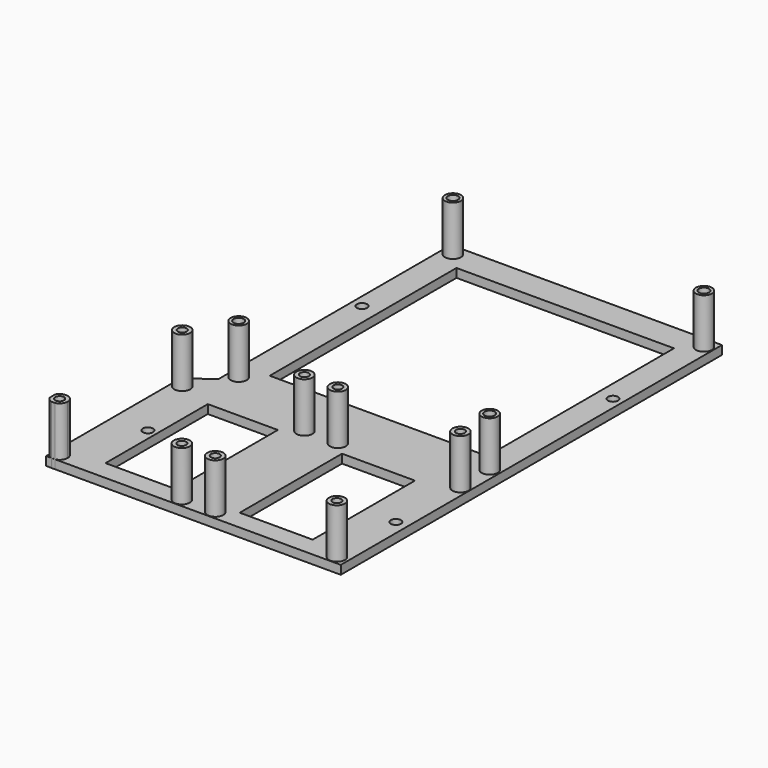
from build123d import *

# Parameters (mm, degrees)
F0_R     = 1.5
F0_R_2   = 1.75
F0_R_3   = 2.75
F0_W     = 24
F0_H     = 43.8174021336
F0_W_2   = 25
F0_W_3   = 74.5545638204
F0_H_2   = 80
F1_DEPTH = 3
F2_DEPTH = 20
F3_DEPTH = 20


# Not quite as in the source:
# - a feature names something its author has since deleted; it is built from what else it names


with BuildPart() as f1:
    # F0 (on Top) → F1 (new body)
    with BuildSketch(Plane.XY):
        with BuildLine():
            ThreePointArc((-47.6736667828, -81.2138915062), (-46.0983603754, -80.2573488478), (-45.4808032601, -78.5209193664))
            ThreePointArc((-45.4808032601, -78.5209193664), (-47.6409939689, -75.8349139681), (-50.7278032601, -77.3687514099))
            Line((-50.7278032601, -77.3687514099), (-50.7278032601, -79.6730873229))
            ThreePointArc((-50.7278032601, -79.6730873229), (-49.9411999358, -80.6742988526), (-48.7879397374, -81.2138915062))
            Line((-48.7879397374, -81.2138915062), (-47.6736667828, -81.2138915062))
        make_face()
        with Locations((-48.2308032601, -78.5209193664)):
            Circle(F0_R, mode=Mode.SUBTRACT)
        with BuildLine():
            ThreePointArc((-50.7278032601, -77.3687514099), (-47.6409939689, -75.8349139681), (-45.4808032601, -78.5209193664))
            ThreePointArc((-45.4808032601, -78.5209193664), (-46.0983603754, -80.2573488478), (-47.6736667828, -81.2138915062))
            Line((-47.6736667828, -81.2138915062), (50.2721967399, -81.2138915062))
            Line((50.2721967399, -81.2138915062), (50.3258705139, 82))
            Line((50.3258705139, 82), (-42.5516068935, 82))
            Line((-42.5516068935, 82), (-42.5516068935, -17.5))
            Line((-42.5516068935, -17.5), (-50.7278032601, -23.6660409719))
            Line((-50.7278032601, -23.6660409719), (-50.7278032601, -77.3687514099))
        make_face()
        with Locations((-38.7351833579, -52.5912989332)):
            Circle(F0_R_2, mode=Mode.SUBTRACT)
        with Locations((-6.5308032601, -78.3)):
            Circle(F0_R_3, mode=Mode.SUBTRACT)
        with Locations((-23.7278032601, -52.5912989332)):
            Rectangle(F0_W, F0_H, mode=Mode.SUBTRACT)
        with Locations((-47.5, -26.9212964922)):
            Circle(F0_R_3, mode=Mode.SUBTRACT)
        with Locations((-38.9970433209, -13.3562097783)):
            Circle(F0_R_3, mode=Mode.SUBTRACT)
        with Locations((-5.8, -26.7)):
            Circle(F0_R_3, mode=Mode.SUBTRACT)
        with Locations((4.9221967399, -78.3)):
            Circle(F0_R_3, mode=Mode.SUBTRACT)
        with Locations((22.7721967399, -52.5912989332)):
            Rectangle(F0_W_2, F0_H, mode=Mode.SUBTRACT)
        with Locations((46.6221967399, -78.3)):
            Circle(F0_R_3, mode=Mode.SUBTRACT)
        with Locations((46.2721967399, -52.5912989332)):
            Circle(F0_R_2, mode=Mode.SUBTRACT)
        with Locations((5.6529477609, -26.7)):
            Circle(F0_R_3, mode=Mode.SUBTRACT)
        with Locations((47.3529477609, -26.2951753209)):
            Circle(F0_R_3, mode=Mode.SUBTRACT)
        with Locations((47.0029571713, -13.3550426021)):
            Circle(F0_R_3, mode=Mode.SUBTRACT)
        with Locations((-38.9970430732, 39.4713241122)):
            Circle(F0_R_2, mode=Mode.SUBTRACT)
        with Locations((-38.7351833579, 78.1026230454)):
            Circle(F0_R_3, mode=Mode.SUBTRACT)
        with Locations((4.2256750166, 32.5)):
            Rectangle(F0_W_3, F0_H_2, mode=Mode.SUBTRACT)
        with Locations((47.0029569268, 39.4713241122)):
            Circle(F0_R_2, mode=Mode.SUBTRACT)
        with Locations((47.2648166418, 78.1026230454)):
            Circle(F0_R_3, mode=Mode.SUBTRACT)
        with BuildLine():
            Line((-50.7278032601, -79.6730873229), (-50.7278032601, -77.3687514099))
            ThreePointArc((-50.7278032601, -77.3687514099), (-50.9808032601, -78.5209193664), (-50.7278032601, -79.6730873229))
        make_face()
        with BuildLine():
            ThreePointArc((-48.7879397374, -81.2138915062), (-48.2308032601, -81.2709193664), (-47.6736667828, -81.2138915062))
            Line((-47.6736667828, -81.2138915062), (-48.7879397374, -81.2138915062))
        make_face()
        with BuildLine():
            ThreePointArc((-48.7879397374, -81.2138915062), (-49.9411999358, -80.6742988526), (-50.7278032601, -79.6730873229))
            Line((-50.7278032601, -79.6730873229), (-50.7278032601, -81.2138915062))
            Line((-50.7278032601, -81.2138915062), (-48.7879397374, -81.2138915062))
        make_face()
    extrude(amount=F1_DEPTH)

    # F0 (on Top) → F2 (join)
    with BuildSketch(Plane.XY):
        with Locations((-38.7351833579, 78.1026230454)):
            Circle(F0_R_3)
        with Locations((-38.7351833579, 78.1026230454)):
            Circle(F0_R_2, mode=Mode.SUBTRACT)
    extrude(amount=F2_DEPTH)

    # F0 (on Top) → F3 (join)
    with BuildSketch(Plane.XY):
        with Locations((47.2648166418, 78.1026230454)):
            Circle(F0_R_3)
        with Locations((47.2648166418, 78.1026230454)):
            Circle(F0_R_2, mode=Mode.SUBTRACT)
        with Locations((-38.9970433209, -13.3562097783)):
            Circle(F0_R_3)
        with Locations((-38.9970433209, -13.3562097783)):
            Circle(F0_R_2, mode=Mode.SUBTRACT)
        with Locations((47.3529477609, -26.2951753209)):
            Circle(F0_R_3)
        with Locations((47.3529477609, -26.2951753209)):
            Circle(F0_R, mode=Mode.SUBTRACT)
        with Locations((5.6529477609, -26.7)):
            Circle(F0_R_3)
        with Locations((5.6529477609, -26.7)):
            Circle(F0_R, mode=Mode.SUBTRACT)
        with Locations((-5.8, -26.7)):
            Circle(F0_R_3)
        with Locations((-5.8, -26.7)):
            Circle(F0_R, mode=Mode.SUBTRACT)
        with Locations((-47.5, -26.9212964922)):
            Circle(F0_R_3)
        with Locations((-47.5, -26.9212964922)):
            Circle(F0_R, mode=Mode.SUBTRACT)
        with BuildLine():
            ThreePointArc((-47.6736667828, -81.2138915062), (-46.0983603754, -80.2573488478), (-45.4808032601, -78.5209193664))
            ThreePointArc((-45.4808032601, -78.5209193664), (-47.6409939689, -75.8349139681), (-50.7278032601, -77.3687514099))
            Line((-50.7278032601, -77.3687514099), (-50.7278032601, -79.6730873229))
            ThreePointArc((-50.7278032601, -79.6730873229), (-49.9411999358, -80.6742988526), (-48.7879397374, -81.2138915062))
            Line((-48.7879397374, -81.2138915062), (-47.6736667828, -81.2138915062))
        make_face()
        with Locations((-48.2308032601, -78.5209193664)):
            Circle(F0_R, mode=Mode.SUBTRACT)
        with Locations((-6.5308032601, -78.3)):
            Circle(F0_R_3)
        with Locations((-6.5308032601, -78.3)):
            Circle(F0_R, mode=Mode.SUBTRACT)
        with Locations((4.9221967399, -78.3)):
            Circle(F0_R_3)
        with Locations((4.9221967399, -78.3)):
            Circle(F0_R, mode=Mode.SUBTRACT)
        with Locations((46.6221967399, -78.3)):
            Circle(F0_R_3)
        with Locations((46.6221967399, -78.3)):
            Circle(F0_R, mode=Mode.SUBTRACT)
        with Locations((47.0029571713, -13.3550426021)):
            Circle(F0_R_3)
        with Locations((47.0029571713, -13.3550426021)):
            Circle(F0_R_2, mode=Mode.SUBTRACT)
    extrude(amount=F3_DEPTH)


solid = f1.part
